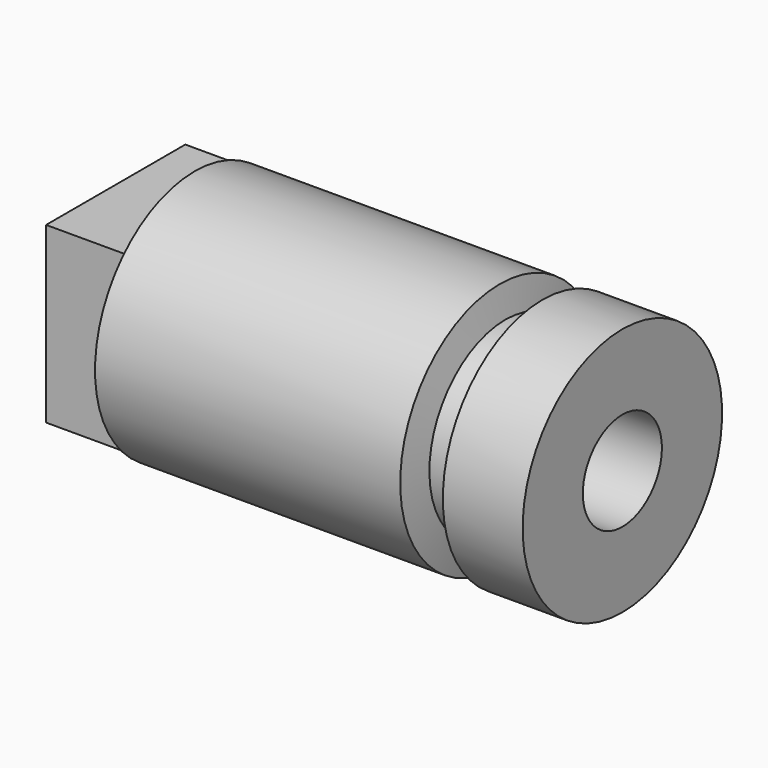
from build123d import *
from build123d import SkipClean  # not in build123d's __all__

# Parameters (mm, degrees)
F2_W     = 17.4498
F2_H     = 17.4498
F2_R     = 4.953
F3_DEPTH = 7.9248


with BuildPart() as f1:
    # F0 (on Front) → F1 (revolve)
    with BuildSketch(Plane.XZ):
        Polygon((1.1196035955, 9.525), (1.1196035955, 4.953), (43.9948035955, 4.953), (43.9948035955, 12.4968), (35.9913689879, 12.4968), (35.4428738503, 9.525), (32.2678738503, 9.525), (31.7193787128, 12.4968), (1.1196035955, 12.4968), align=None)
    revolve(axis=Axis((1.9816491438, 0, 0), (1, 0, 0)))

    # F2 (on face) → F3 (join)
    with BuildSketch(Plane(origin=(1.1196035955, 0, 0), x_dir=(0, -1, 0), z_dir=(-1, 0, 0))):
        Rectangle(F2_W, F2_H)
        Circle(F2_R, mode=Mode.SUBTRACT)
    with SkipClean():  # cleaning this boolean's faces spoils the solid; the shape is the same uncleaned
        extrude(amount=F3_DEPTH)


solid = f1.part
